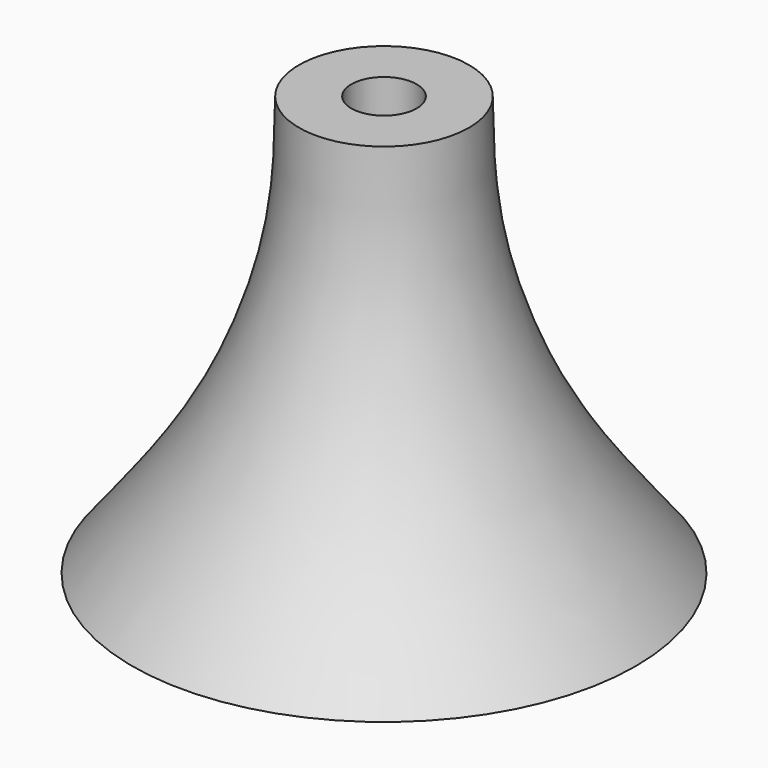
from build123d import *

# Parameters (mm, degrees)
F2_R     = 7.7938350574
F3_DEPTH = 100


with BuildPart() as f1:
    # F0 (on Front) → F1 (revolve)
    with BuildSketch(Plane.XZ):
        with BuildLine():
            Line((20.2545374632, 49.4481252445), (0, 49.4481252445))
            Line((0, 49.4481252445), (0, -50.5518747555))
            Line((0, -50.5518747555), (60, -50.5518747555))
            add(Edge.make_bspline(
                [(20.2545374632, 49.4481252445), (20.384835388, 40.1210020342), (20.6673970939, 19.8943725713), (34.3036697283, -18.3289138464), (51.3680245863, -39.7274572848), (60, -50.5518747555)],
                knots=[0, 0, 0, 0, 0.2971923548, 0.6444859261, 1, 1, 1, 1], degree=3))
        make_face()
    revolve(axis=Axis((0, 0, -0.5518747555), (0, 0, -1)))

    # F2 (on Top) → F3 (cut)
    with BuildSketch(Plane.XY):
        Circle(F2_R)
    extrude(amount=F3_DEPTH, mode=Mode.SUBTRACT)


solid = f1.part
